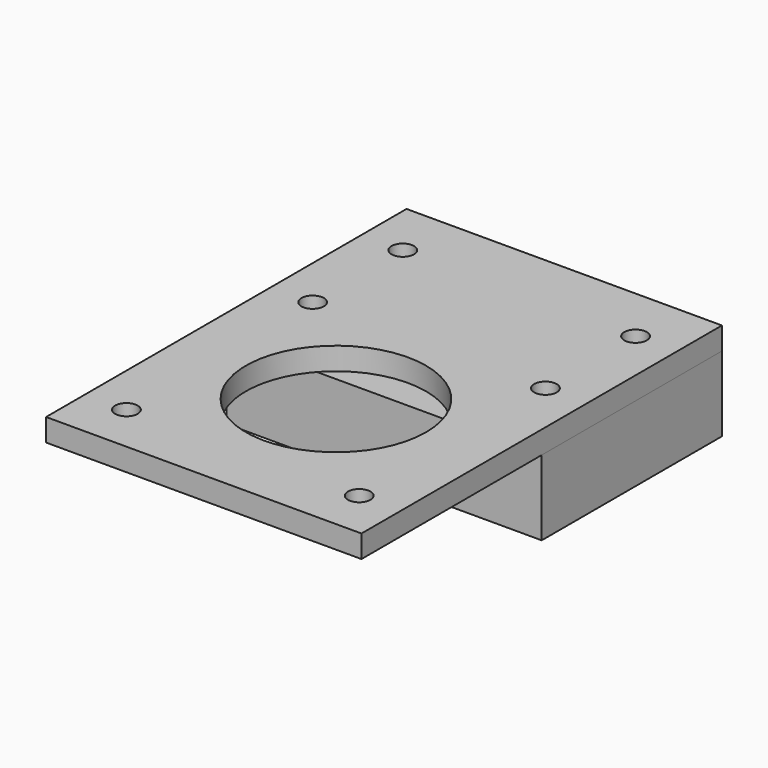
from build123d import *

# Parameters (mm, degrees)
F0_W     = 42
F0_H     = 30
F1_DEPTH = 10
F2_DEPTH = 3
F3_DEPTH = 30
F5_D     = 3
F5_2_D   = 3
F4_R     = 12
F6_DEPTH = 25


with BuildPart() as f1:
    # F0 (on Top) → F1 (new body)
    with BuildSketch(Plane.XY):
        Rectangle(F0_W, F0_H)
    extrude(amount=F1_DEPTH)


with BuildPart() as f2:
    # F2 (new): a face of the model
    f2_faces = [f1.part.faces().sort_by_distance(p)[0] for p in [
        (0, 0, 10),
    ]]
    extrude(f2_faces, amount=F2_DEPTH)

    # F3 (add): a face of the model
    f3_faces = [f2.faces().sort_by_distance(p)[0] for p in [
        (0, -15, 11.5),
    ]]
    extrude(f3_faces, amount=F3_DEPTH)

    # F5#2 (through all)
    with Locations(Plane.XY.offset(13)):
        with Locations((-15.5, -7.5), (-15.5, 7.5), (15.5, 7.5), (15.5, -7.5), (15.5, -38.5), (-15.5, -38.5)):
            Hole(F5_2_D / 2)

    # F4 (on face) → F6 (cut)
    with BuildSketch(Plane.XY.offset(13)):
        with Locations((0, -23)):
            Circle(F4_R)
    extrude(amount=-F6_DEPTH, mode=Mode.SUBTRACT)


with BuildPart() as f1_1:
    add(f1.part)

    # F5 (through all)
    with Locations(Plane.XY.offset(13)):
        with Locations((-15.5, -7.5), (-15.5, 7.5), (15.5, 7.5), (15.5, -7.5), (15.5, -38.5), (-15.5, -38.5)):
            Hole(F5_D / 2)


solid = Compound([f2.part, f1_1.part])
